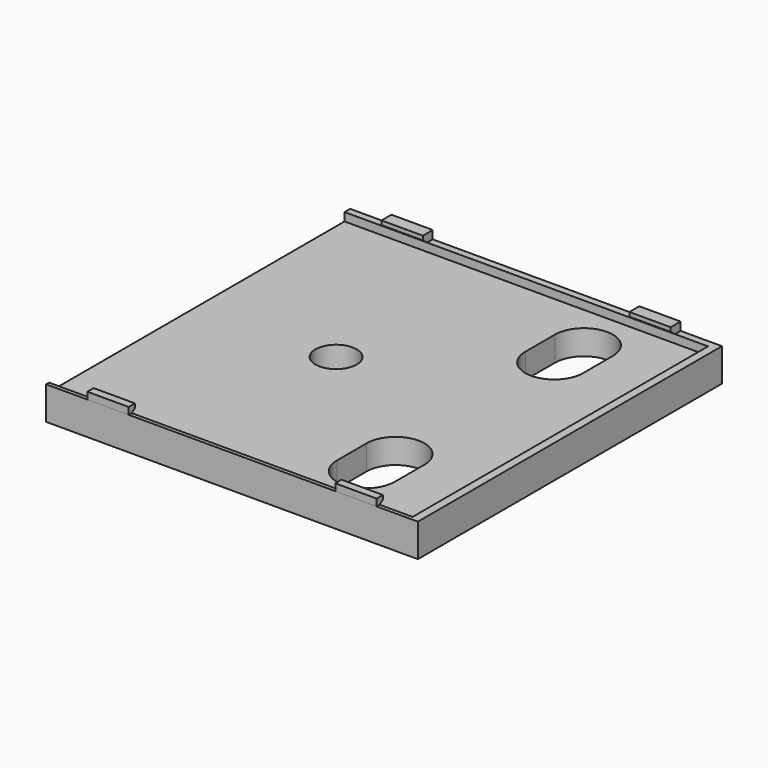
from build123d import *

# Parameters (mm, degrees)
F0_W     = 45
F0_H     = 46
F0_R     = 2.5
F1_DEPTH = 4
F2_W     = 44
F2_H     = 44.7
F2_R     = 2.5
F3_DEPTH = 1
F5_DEPTH = 5
F6_DEPTH = 5


# Not quite as in the source:
# - a feature names something its author has since deleted; it is built from what else it names


with BuildPart() as f1:
    # F0 (on Top) → F1 (new body)
    with BuildSketch(Plane.XY):
        with Locations((22.5, 23)):
            Rectangle(F0_W, F0_H)
        with BuildLine():
            ThreePointArc((37, 6.5), (33.5, 3), (30, 6.5))
            Line((30, 6.5), (30, 11))
            ThreePointArc((30, 11), (33.5, 14.5), (37, 11))
            Line((37, 11), (37, 6.5))
        make_face(mode=Mode.SUBTRACT)
        with Locations((16.7, 23)):
            Circle(F0_R, mode=Mode.SUBTRACT)
        with BuildLine():
            Line((30, 35), (30, 39.5))
            ThreePointArc((30, 39.5), (33.5, 43), (37, 39.5))
            Line((37, 39.5), (37, 35))
            ThreePointArc((37, 35), (33.5, 31.5), (30, 35))
        make_face(mode=Mode.SUBTRACT)
    extrude(amount=F1_DEPTH)

    # F2 (on face) → F3 (cut)
    with BuildSketch(Plane.XY.offset(4)):
        with Locations((22, 22.8)):
            Rectangle(F2_W, F2_H)
        with BuildLine():
            Line((37, 11), (37, 6.5))
            ThreePointArc((37, 6.5), (33.5, 3), (30, 6.5))
            Line((30, 6.5), (30, 11))
            ThreePointArc((30, 11), (33.5, 14.5), (37, 11))
        make_face(mode=Mode.SUBTRACT)
        with Locations((16.7, 23)):
            Circle(F2_R, mode=Mode.SUBTRACT)
        with BuildLine():
            ThreePointArc((37, 35), (33.5, 31.5), (30, 35))
            Line((30, 35), (30, 39.5))
            ThreePointArc((30, 39.5), (33.5, 43), (37, 39.5))
            Line((37, 39.5), (37, 35))
        make_face(mode=Mode.SUBTRACT)
    extrude(amount=-F3_DEPTH, mode=Mode.SUBTRACT)


with BuildPart() as f5:
    # F4 (on face) → F5 (new body)
    with BuildSketch(Plane(origin=(0, 0, 0), x_dir=(0, -1, 0), z_dir=(-1, 0, 0))):
        Polygon((-46, 4), (-45.15, 4), (-44.5, 4.5), (-44.5, 5), (-46, 5), align=None)
    extrude(amount=-F5_DEPTH)


with BuildPart() as f6:
    # F4 (on face) → F6 (new body)
    with BuildSketch(Plane(origin=(0, 0, 0), x_dir=(0, -1, 0), z_dir=(-1, 0, 0))):
        Polygon((-0.95, 4.3347524479), (-0.45, 4), (0, 4), (0, 4.8347524479), (-0.95, 4.8347524479), align=None)
    extrude(amount=-F6_DEPTH)


with BuildPart() as f7_1:
    # F7: copy of F6
    add(f6.part.moved(Location((40, 0, 0))))


with BuildPart() as f8_1:
    # F8: copy of F5
    add(f5.part.moved(Location((40, 0, 0))))


with BuildPart() as f5_1:
    # F9: moved
    add(f5.part.moved(Location((5, 0, 0))))


with BuildPart() as f6_1:
    # F9: moved
    add(f6.part.moved(Location((5, 0, 0))))


with BuildPart() as f7_1_1:
    # F10: moved
    add(f7_1.part.moved(Location((-5, 0, 0))))


with BuildPart() as f8_1_1:
    # F10: moved
    add(f8_1.part.moved(Location((-5, 0, 0))))


solid = Compound([f1.part, f5_1.part, f6_1.part, f7_1_1.part, f8_1_1.part])
